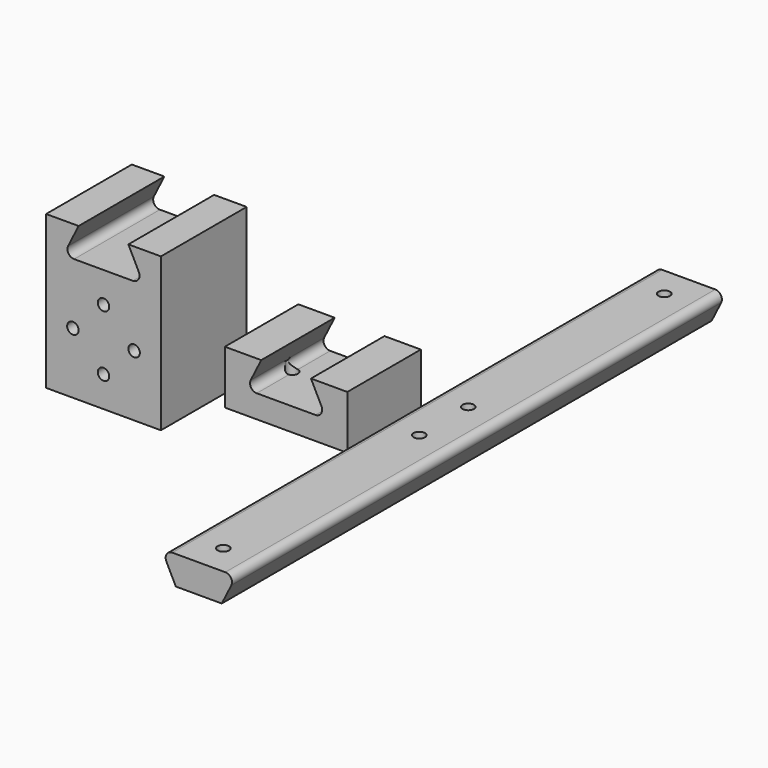
from build123d import *

# Parameters (mm, degrees)
F1_DEPTH      = 12
F3_DEPTH      = 80
F4_R          = 1.5
F5_DEPTH      = 7
F6_R          = 1.5
F7_DEPTH      = 13.9952990129
F9_DEPTH      = 28
F10_T4_DEPTH  = 24
F10_S5_R      = 1.5
F10_T6_DEPTH  = 14
F10_T10_DEPTH = 24
F10_S11_R     = 1.5
F10_T12_DEPTH = 14
F10_2_F1_R    = 1.75
F10_2_F2_R    = 1.75
F10_3_F1_R    = 1.75
F10_3_F2_R    = 1.75
F11_R         = 1.5
F12_DEPTH     = 108.001


# Not quite as in the source:
# - a fillet or chamfer that OpenCascade refuses, or shapes differently, is made with other operations: its cross-section is extruded or revolved along the edge and cut away or added


with BuildPart() as f1:
    # F0 (on Front) → F1 (new body, symmetric)
    with BuildSketch(Plane.XZ):
        Polygon((19.5705028659, -0.0057009871), (19.5705028659, 13.9942990129), (10.0705028659, 13.9942990129), (14.0705028659, 5.9942990129), (-6.9294971341, 5.9942990129), (-2.9294971341, 13.9942990129), (-12.4294971341, 13.9942990129), (-12.4294971341, -0.0057009871), align=None)
    extrude(amount=F1_DEPTH, both=True)

    # F4 (on face) → F5 (cut)
    with BuildSketch(Plane(origin=(0, 0, -0.0057009871), x_dir=(1, 0, 0), z_dir=(0, 0, -1))):
        with Locations((-4.4294971341, 0)):
            Circle(F4_R)
        with Locations((11.5705028659, 0)):
            Circle(F4_R)
    extrude(amount=-F5_DEPTH, mode=Mode.SUBTRACT)

    # F10: fillet of radius 1.75 on 2 edges, made by hand


with BuildPart() as f3:
    # F2 (on Front) → F3 (new body, symmetric)
    with BuildSketch(Plane.XZ):
        Polygon((25.415773809, 7.5), (29.165773809, 0), (41.165773809, 0), (44.915773809, 7.5), align=None)
    extrude(amount=F3_DEPTH, both=True)

    # F6 (on face) → F7 (cut, through all)
    with BuildSketch(Plane(origin=(0, 0, 0), x_dir=(1, 0, 0), z_dir=(0, 0, -1))):
        with Locations((35.165773809, 72)):
            Circle(F6_R)
        with Locations((35.165773809, -72)):
            Circle(F6_R)
        with Locations((35.165773809, 8)):
            Circle(F6_R)
        with Locations((35.165773809, -8)):
            Circle(F6_R)
    extrude(amount=-F7_DEPTH, mode=Mode.SUBTRACT)

    # F10#2: fillet of radius 1.75 on 2 edges, made by hand

    # F10_2_f1
    f10_2_f1_edges = [f3.edges().sort_by_distance(p)[0] for p in [
        (44.915773809, 0, 7.5),
    ]]
    fillet(f10_2_f1_edges, radius=F10_2_F1_R)

    # F10_2_f2
    f10_2_f2_edges = [f3.edges().sort_by_distance(p)[0] for p in [
        (25.415773809, 0, 7.5),
    ]]
    fillet(f10_2_f2_edges, radius=F10_2_F2_R)


with BuildPart() as f9:
    # F8 (on Front) → F9 (new body)
    with BuildSketch(Plane.XZ):
        Polygon((-46.3340594471, 40), (-46.3340594471, 0), (-16.3340594471, 0), (-16.3340594471, 40), (-24.8340594471, 40), (-20.8340594471, 32), (-41.8340594471, 32), (-37.8340594471, 40), align=None)
    extrude(amount=F9_DEPTH)

    # F10#3: fillet of radius 1.75 on 2 edges, made by hand

    # F10_3_f1
    f10_3_f1_edges = [f9.edges().sort_by_distance(p)[0] for p in [
        (-20.8340594471, -14, 32),
    ]]
    fillet(f10_3_f1_edges, radius=F10_3_F1_R)

    # F10_3_f2
    f10_3_f2_edges = [f9.edges().sort_by_distance(p)[0] for p in [
        (-41.8340594471, -14, 32),
    ]]
    fillet(f10_3_f2_edges, radius=F10_3_F2_R)

    # F11 (on face) → F12 (cut, through all)
    with BuildSketch(Plane.XZ.offset(28)):
        with Locations((-31.3340594471, 24)):
            Circle(F11_R)
        with Locations((-23.3340594471, 16)):
            Circle(F11_R)
        with Locations((-31.3340594471, 8)):
            Circle(F11_R)
        with Locations((-39.3340594471, 16)):
            Circle(F11_R)
    extrude(amount=-F12_DEPTH, mode=Mode.SUBTRACT)


with BuildPart() as f10_tool2:
    # F10_s3 → F10_t4 (new body)
    with BuildSketch(Plane.XZ.offset(-12)):
        with BuildLine():
            ThreePointArc((-4.0979376538, 5.9942990129), (-5.5865765684, 6.8242695667), (-5.663185238, 8.5269228051))
            Line((-5.663185238, 8.5269228051), (-6.9294971341, 5.9942990129))
            Line((-6.9294971341, 5.9942990129), (-4.0979376538, 5.9942990129))
        make_face()
    extrude(amount=F10_T4_DEPTH)

    # F10_s5 → F10_t6 (cut, symmetric)
    with BuildSketch(Plane.XY.offset(7.3)):
        with Locations((-4.4294971341, 0)):
            Circle(F10_S5_R)
    extrude(amount=F10_T6_DEPTH, both=True, mode=Mode.SUBTRACT)


with BuildPart() as f1_1:
    add(f1.part)

    # F10_t1: union F10_tool2
    add(f10_tool2.part)


with BuildPart() as f10_tool8:
    # F10_s9 → F10_t10 (new body)
    with BuildSketch(Plane.XZ.offset(-12)):
        with BuildLine():
            ThreePointArc((12.8041909699, 8.5269228051), (12.7275823002, 6.8242695667), (11.2389433856, 5.9942990129))
            Line((11.2389433856, 5.9942990129), (14.0705028659, 5.9942990129))
            Line((14.0705028659, 5.9942990129), (12.8041909699, 8.5269228051))
        make_face()
    extrude(amount=F10_T10_DEPTH)

    # F10_s11 → F10_t12 (cut, symmetric)
    with BuildSketch(Plane.XY.offset(7.3)):
        with Locations((11.5705028659, 0)):
            Circle(F10_S11_R)
    extrude(amount=F10_T12_DEPTH, both=True, mode=Mode.SUBTRACT)


with BuildPart() as f1_2:
    add(f1_1.part)

    # F10_t7: union F10_tool8
    add(f10_tool8.part)


solid = Compound([f3.part, f9.part, f1_2.part])
